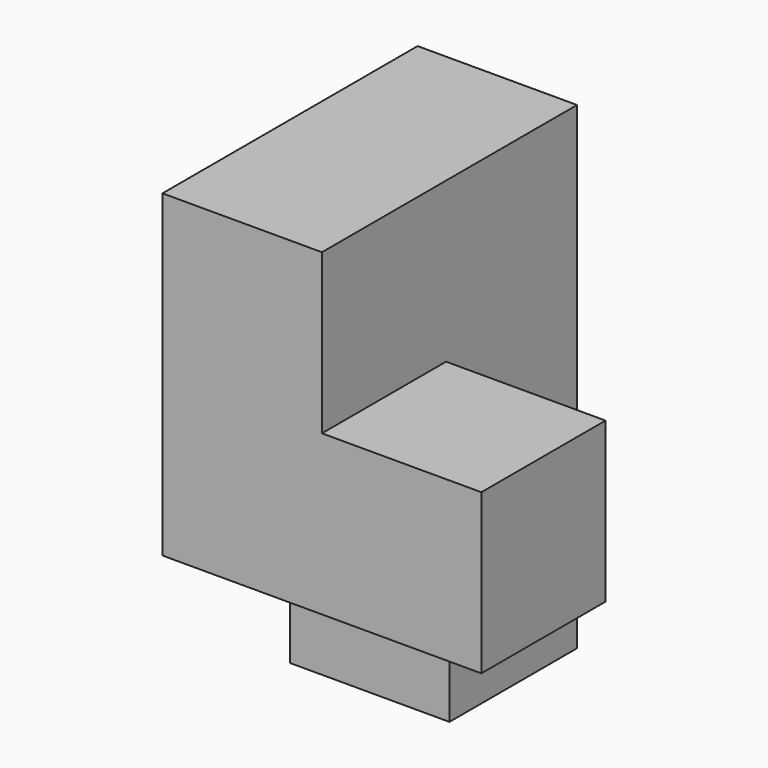
from build123d import *

# Parameters (mm, degrees)
F0_W     = 19.05
F0_H     = 19.05
F1_DEPTH = 57.15
F2_W     = 19.05
F2_H     = 38.1
F3_DEPTH = 19.05
F4_W     = 18.542
F4_H     = 19.05
F5_DEPTH = 19.05


# Not quite as in the source:
# - a feature names something its author has since deleted; it is built from what else it names


with BuildPart() as f1:
    # F0 (on Top) → F1 (new body)
    with BuildSketch(Plane.XY):
        with Locations((9.525, -9.525)):
            Rectangle(F0_W, F0_H)
    extrude(amount=F1_DEPTH)

    # F2 (on face) → F3 (join)
    with BuildSketch(Plane.XZ.offset(19.05)):
        with Locations((9.525, 38.1)):
            Rectangle(F2_W, F2_H)
    extrude(amount=F3_DEPTH)

    # F4 (on face) → F5 (join)
    with BuildSketch(Plane.YZ.offset(19.05)):
        with Locations((-28.829, 28.575)):
            Rectangle(F4_W, F4_H)
    extrude(amount=F5_DEPTH)


solid = f1.part
